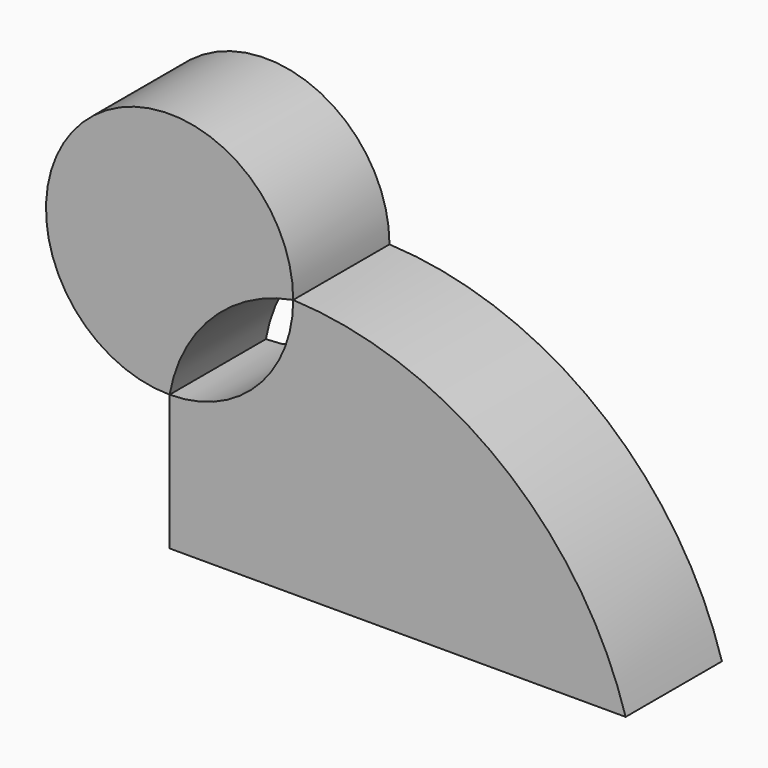
from build123d import *

# Parameters (mm, degrees)
F1_DEPTH    = 25.4
F2_T1_DEPTH = 408.305123953
F3_T1_DEPTH = 25.4


# Not quite as in the source:
# - a fillet or chamfer that OpenCascade refuses, or shapes differently, is made with other operations: its cross-section is extruded or revolved along the edge and cut away or added


with BuildPart() as f1:
    # F0 (on Front) → F1 (new body)
    with BuildSketch(Plane.XZ):
        with BuildLine():
            ThreePointArc((-23.6390728491, 27.3305587471), (-68.1810033514, 45.7804304554), (-49.7311316431, 1.2384999531))
            Line((-49.7311316431, 1.2384999531), (-49.7311316431, 27.3305587471))
            Line((-49.7311316431, 27.3305587471), (-23.6390728491, 27.3305587471))
        make_face()
    extrude(amount=F1_DEPTH)

    # F3: fillet of radius 32.1935378542 on 1 edges, made by hand

    # F3_s2 → F3_t1 (join)
    with BuildSketch(Plane.XZ):
        with BuildLine():
            ThreePointArc((-49.7311316431, 1.2384999531), (-40.7942631124, 18.3936902164), (-23.6390728491, 27.3305587471))
            Line((-23.6390728491, 27.3305587471), (-49.7311316431, 27.3305587471))
            Line((-49.7311316431, 27.3305587471), (-49.7311316431, 1.2384999531))
        make_face()
    extrude(amount=F3_T1_DEPTH)


with BuildPart() as f1b:
    # F0 (on Front) → F1, piece 2 (new body)
    with BuildSketch(Plane.XZ):
        with BuildLine():
            Line((-49.7311316431, -27.3305587471), (49.7311316431, -27.3305587471))
            Line((49.7311316431, -27.3305587471), (49.7311316431, 27.3305587471))
            Line((49.7311316431, 27.3305587471), (-23.6390728491, 27.3305587471))
            ThreePointArc((-23.6390728491, 27.3305587471), (-31.2812599347, 8.8806870387), (-49.7311316431, 1.2384999531))
            Line((-49.7311316431, 1.2384999531), (-49.7311316431, -27.3305587471))
        make_face()
    extrude(amount=F1_DEPTH)

    # F2: fillet of radius 76.6512806053 on 1 edges, made by hand

    # F2_s2 → F2_t1 (cut)
    with BuildSketch(Plane.XZ.offset(-191.4525619765)):
        with BuildLine():
            ThreePointArc((49.7311316431, -49.2504660436), (28.4283718141, 3.7774517574), (-23.6390728491, 27.3305587471))
            Line((-23.6390728491, 27.3305587471), (49.7311316431, 27.3305587471))
            Line((49.7311316431, 27.3305587471), (49.7311316431, -49.2504660436))
        make_face()
    extrude(amount=F2_T1_DEPTH, mode=Mode.SUBTRACT)


solid = Compound([f1.part, f1b.part])
